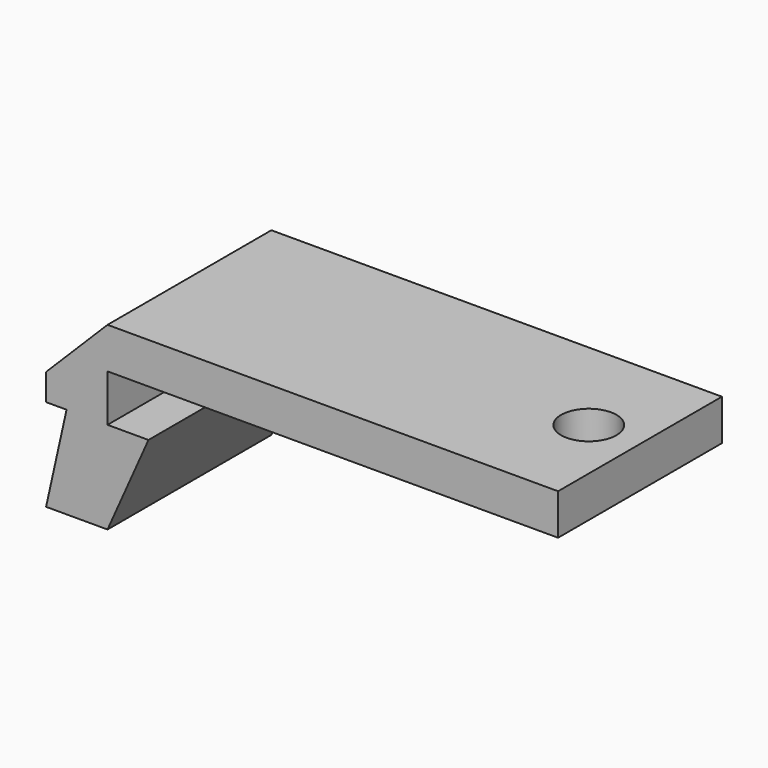
from build123d import *

# Parameters (mm, degrees)
F1_DEPTH = 10
F2_R     = 1.35
F3_DEPTH = 25


# Not quite as in the source:
# - a feature names something its author has since deleted; it is built from what else it names


with BuildPart() as f1:
    # F0 (on Front) → F1 (new body)
    with BuildSketch(Plane.XZ):
        Polygon((-3, 0), (0, 0), (2, 4.5), (0, 4.5), (0, 6.8), (22, 6.8), (22, 8.8), (0, 8.8), (-3, 5.8), (-3, 4.5), (-2, 4.5), align=None)
    extrude(amount=F1_DEPTH)

    # F2 (on face) → F3 (cut)
    with BuildSketch(Plane.XY.offset(8.8)):
        with Locations((19.5, -5)):
            Circle(F2_R)
    extrude(amount=-F3_DEPTH, mode=Mode.SUBTRACT)


solid = f1.part
